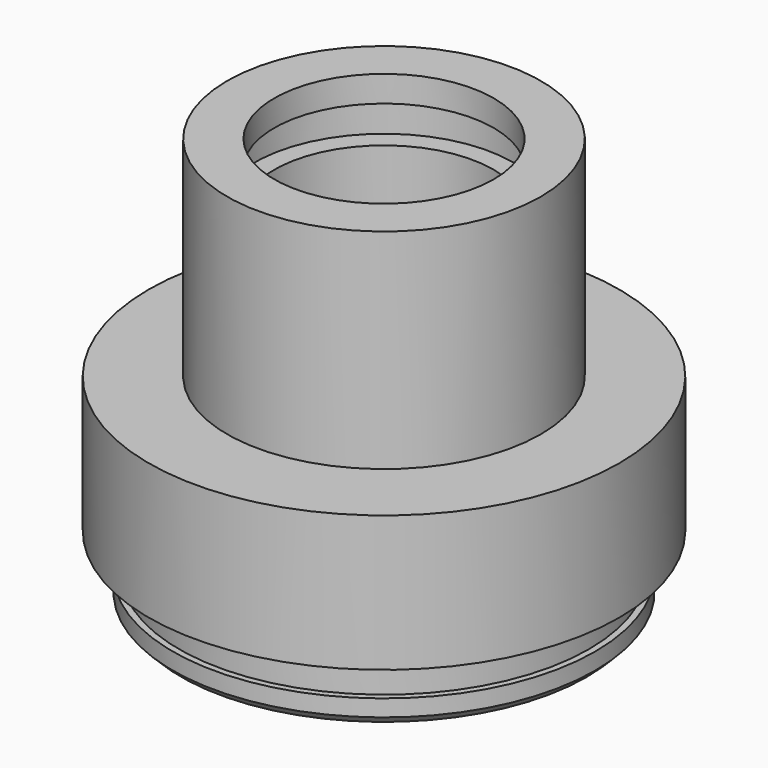
from build123d import *

# Parameters (mm, degrees)
F0_R           = 9.525
F1_DEPTH       = 12.7
F2_R           = 6.6675
F3_DEPTH       = 9.525
F4_W           = 1.1938
F4_H           = 2.2352
F6_R           = 14.2875
F6_R_2         = 9.525
F7_DEPTH       = 8.255
F8_R           = 12.827
F9_DEPTH       = 3.81
F10_R          = 10.2235
F11_DEPTH      = 3.81
F12_W          = 0.381
F12_H          = 2.286
F14_R          = 2.6035
F15_DEPTH      = 25.4
F15_DEPTH_BACK = 25.4
F16_SIZE       = 0.508


with BuildPart() as f1:
    # F0 (on Top) → F1 (new body)
    with BuildSketch(Plane.XY):
        Circle(F0_R)
    extrude(amount=F1_DEPTH)

    # F2 (on face) → F3 (cut)
    with BuildSketch(Plane.XY.offset(12.7)):
        Circle(F2_R)
    extrude(amount=-F3_DEPTH, mode=Mode.SUBTRACT)

    # F4 (on Front) → F5 (revolve, cut)
    with BuildSketch(Plane.XZ):
        with Locations((7.2644, 9.9949)):
            Rectangle(F4_W, F4_H)
    revolve(axis=Axis((0, 0, 19.0221574157), (0, 0, 1)), mode=Mode.SUBTRACT)

    # F6 (on face) → F7 (join)
    with BuildSketch(Plane(origin=(0, 0, 0), x_dir=(1, 0, 0), z_dir=(0, 0, -1))):
        Circle(F6_R)
        Circle(F6_R_2, mode=Mode.SUBTRACT)
        Circle(F6_R_2)
    extrude(amount=F7_DEPTH)

    # F8 (on face) → F9 (join)
    with BuildSketch(Plane(origin=(0, 0, -8.255), x_dir=(1, 0, 0), z_dir=(0, 0, -1))):
        Circle(F8_R)
    extrude(amount=F9_DEPTH)

    # F10 (on face) → F11 (cut)
    with BuildSketch(Plane(origin=(0, 0, -12.065), x_dir=(1, 0, 0), z_dir=(0, 0, -1))):
        Circle(F10_R)
    extrude(amount=-F11_DEPTH, mode=Mode.SUBTRACT)

    # F12 (on Front) → F13 (revolve, cut)
    with BuildSketch(Plane.XZ):
        with Locations((12.6365, -9.398)):
            Rectangle(F12_W, F12_H)
    revolve(axis=Axis((0, 0, -8.9314272627), (0, 0, -1)), mode=Mode.SUBTRACT)

    # F14 (on face) → F15 (cut, two sides)
    with BuildSketch(Plane.XY.offset(3.175)) as f15_sk:
        Circle(F14_R)
    extrude(amount=-F15_DEPTH, mode=Mode.SUBTRACT)
    extrude(f15_sk.sketch, amount=F15_DEPTH_BACK, mode=Mode.SUBTRACT)

    # F16
    f16_edges = [f1.edges().sort_by_distance(p)[0] for p in [
        (-10.2235, 0, -12.065),
        (-12.827, 0, -12.065),
    ]]
    chamfer(f16_edges, length=F16_SIZE)


solid = f1.part
